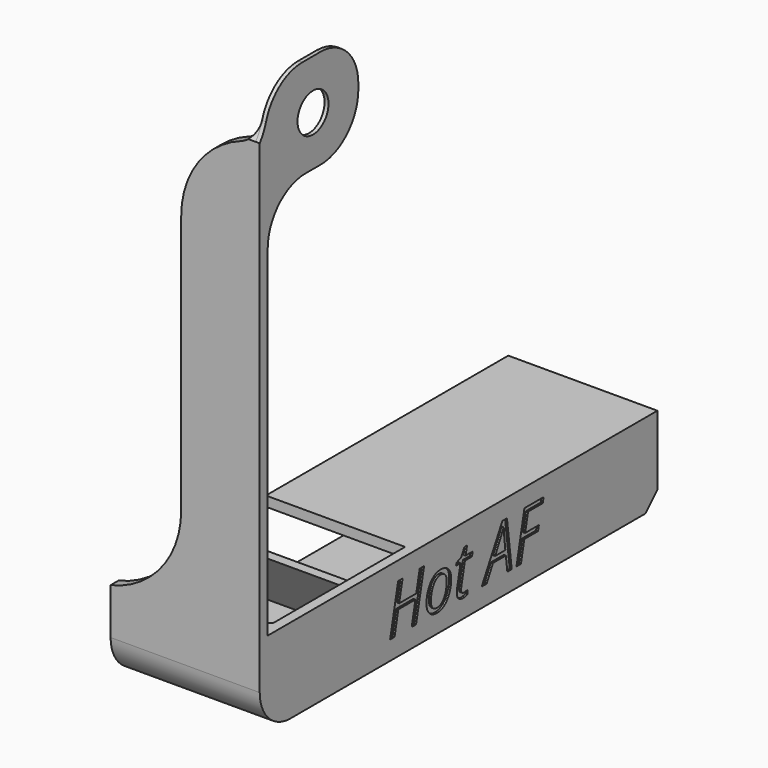
from build123d import *

# Parameters (mm, degrees)
F0_R          = 1.95
F0_W          = 30.45
F0_H          = 8.5
F1_DEPTH      = 0.4
F2_DEPTH      = 14.6
F3_T1_DEPTH   = 0.4
F4_R          = 4.7560007179
F5_R          = 3.8627416998
F6_SIZE       = 1.5
F7_DEPTH      = 7.5
F8_T1_DEPTH   = 1
F8_T3_DEPTH   = 46.0999370995
F9_T4_DEPTH   = 1
F9_S5_R       = 4.9999999991
F9_T6_DEPTH   = 3
F12_DEPTH     = 14
F13_C1_SIZE   = 2
F13_C2_SIZE   = 2
F13_C3_SIZE   = 2
F10_TEXT_SIZE = 6.6774479629
F14_DEPTH     = 0.2


# Not quite as in the source:
# - a fillet or chamfer that OpenCascade refuses, or shapes differently, is made with other operations: its cross-section is extruded or revolved along the edge and cut away or added
# - Text() gives the source's letters only with a copy of the font that has no kerning and outlines rounded to 1/6400 em; it was checked with that copy


with BuildPart() as f1:
    # F0 (on Right) → F1 (new body)
    with BuildSketch(Plane.YZ):
        Polygon((5.7, -5), (5.7, 5), (-5.7, 5), (-5.7, 0), (-5.7, -5), align=None)
        Circle(F0_R, mode=Mode.SUBTRACT)
        Polygon((-5.7, -5), (-5.7, 0), (-6.7, 0), (-6.7, -44), (-5.7, -44), align=None)
        Polygon((12.85, -44), (-5.7, -44), (-6.7, -44), (-6.7, -52.5), (12.85, -52.5), align=None)
        with Locations((28.075, -48.25)):
            Rectangle(F0_W, F0_H)
    extrude(amount=F1_DEPTH)

    # F0 (on Right) → F2 (join)
    with BuildSketch(Plane.YZ):
        Polygon((12.85, -44), (-5.7, -44), (-6.7, -44), (-6.7, -52.5), (12.85, -52.5), align=None)
        with Locations((28.075, -48.25)):
            Rectangle(F0_W, F0_H)
    extrude(amount=-F2_DEPTH)

    # F3: fillet of radius 5 on 1 edges, made by hand

    # F3_s2 → F3_t1 (join)
    with BuildSketch(Plane.YZ):
        with BuildLine():
            ThreePointArc((-6.7, 0), (-5.9565835097, 1.4188611699), (-5.7, 3))
            Line((-5.7, 3), (-5.7, 0))
            Line((-5.7, 0), (-6.7, 0))
        make_face()
    extrude(amount=F3_T1_DEPTH)

    # F4
    f4_edges = [f1.edges().sort_by_distance(p)[0] for p in [
        (0.2, -5.7, 5),
        (0.2, 5.7, 5),
        (0.2, 5.7, -5),
        (0.2, -5.7, -5),
    ]]
    fillet(f4_edges, radius=F4_R)

    # F5
    f5_edges = [f1.edges().sort_by_distance(p)[0] for p in [
        (-7.1, -6.7, -52.5),
    ]]
    fillet(f5_edges, radius=F5_R)

    # F6
    f6_edges = [f1.edges().sort_by_distance(p)[0] for p in [
        (-7.1, 43.3, -52.5),
    ]]
    chamfer(f6_edges, length=F6_SIZE)

    # F0 (on Right) → F7 (join)
    with BuildSketch(Plane.YZ):
        Polygon((-5.7, -5), (-5.7, 0), (-6.7, 0), (-6.7, -44), (-5.7, -44), align=None)
    extrude(amount=-F7_DEPTH)

    # F8: fillet of radius 9.174011537 on 2 edges, made by hand

    # F8_s2 → F8_t1 (join)
    with BuildSketch(Plane.XZ.offset(5.7)):
        with BuildLine():
            ThreePointArc((-7.5, -35.0635038284), (-9.4910632061, -40.7703191361), (-14.6, -44))
            Line((-14.6, -44), (-7.5, -44))
            Line((-7.5, -44), (-7.5, -35.0635038284))
        make_face()
    extrude(amount=F8_T1_DEPTH)

    # F8_s4 → F8_t3 (cut)
    with BuildSketch(Plane.XZ.offset(-16.8499685498)):
        with BuildLine():
            ThreePointArc((0, 0), (-5.3800613587, -3.154619293), (-7.5, -9.0199874199))
            Line((-7.5, -9.0199874199), (-7.5, 0))
            Line((-7.5, 0), (0, 0))
        make_face()
    extrude(amount=F8_T3_DEPTH, mode=Mode.SUBTRACT)

    # F9: fillet of radius 2.1628679683 on 1 edges, made by hand


with BuildPart() as f9_tool2:
    # F9_s3 → F9_t4 (new body)
    with BuildSketch(Plane.XZ.offset(5.7)):
        with BuildLine():
            ThreePointArc((0, 1.6478704991), (-0.3935135421, 0.4039320911), (-1.4308619718, -0.3873604631))
            ThreePointArc((-1.4308619718, -0.3873604631), (-0.7232676712, -0.1647324784), (0, 0))
            Line((0, 0), (0, 1.6478704991))
        make_face()
    extrude(amount=F9_T4_DEPTH)

    # F9_s5 → F9_t6 (cut, symmetric)
    with BuildSketch(Plane.YZ.offset(-0.7)):
        with Locations((-10.6999999991, 2.9999999997)):
            Circle(F9_S5_R)
    extrude(amount=F9_T6_DEPTH, both=True, mode=Mode.SUBTRACT)


with BuildPart() as f1_1:
    add(f1.part)

    # F9_t1: union F9_tool2
    add(f9_tool2.part)

    # F11 (on face) → F12 (cut)
    with BuildSketch(Plane(origin=(-14.6, 0, 0), x_dir=(0, -1, 0), z_dir=(-1, 0, 0))):
        with BuildLine():
            Line((-12.8277624026, -44), (-12.8277624026, -45))
            Line((-12.8277624026, -45), (-42.3, -45))
            Line((-42.3, -45), (-42.3, -50.5857864376))
            Line((-42.3, -50.5857864376), (-41.3857864376, -51.5))
            Line((-41.3857864376, -51.5), (-11.3289048895, -51.5))
            Line((-11.3289048895, -51.5), (-7.7518734863, -45.4829536864))
            Line((-7.7518734863, -45.4829536864), (-6.7518734863, -45.4829536864))
            Line((-6.7518734863, -45.4829536864), (-10.3289048895, -51.5))
            Line((-10.3289048895, -51.5), (2.8372583002, -51.5))
            ThreePointArc((2.8372583002, -51.5), (4.8615223689, -50.6615223689), (5.7, -48.6372583002))
            Line((5.7, -48.6372583002), (5.7, -45))
            Line((5.7, -45), (5.7, -44))
            Line((5.7, -44), (-12.8277624026, -44))
        make_face()
    extrude(amount=-F12_DEPTH, mode=Mode.SUBTRACT)

    # F13: chamfer of 2 on 6 edges, made by hand

    # F13_c1
    f13_c1_edges = [f1_1.edges().sort_by_distance(p)[0] for p in [
        (-0.6, 42.3, -47.7928932188),
    ]]
    chamfer(f13_c1_edges, length=F13_C1_SIZE)

    # F13_c2
    f13_c2_edges = [f1_1.edges().sort_by_distance(p)[0] for p in [
        (-0.6, 25.8144524448, -51.5),
    ]]
    chamfer(f13_c2_edges, length=F13_C2_SIZE)

    # F13_c3
    f13_c3_edges = [f1_1.edges().sort_by_distance(p)[0] for p in [
        (-0.6, -5.7, -46.3186291501),
        (-0.6, 3.7458232947, -51.5),
        (-0.6, -4.8615223689, -50.6615223689),
    ]]
    chamfer(f13_c3_edges, length=F13_C3_SIZE)

    # F10 (on face) → F14 (cut)
    with BuildSketch(Plane.YZ.offset(0.4)):
        with Locations((9.4169946387, -50.6000071764)):
            Text('Hot AF', F10_TEXT_SIZE, font='Open Sans', font_style=FontStyle.ITALIC, text_align=(TextAlign.LEFT, TextAlign.BOTTOM))
    extrude(amount=-F14_DEPTH, mode=Mode.SUBTRACT)


solid = f1_1.part
